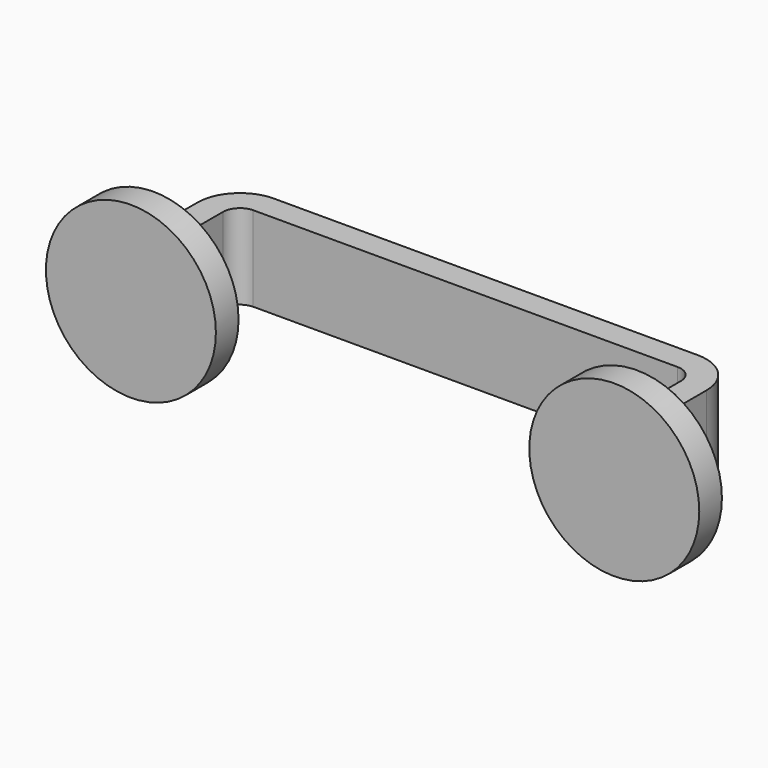
from build123d import *

# Parameters (mm, degrees)
F1_DEPTH = 30
F2_R     = 30
F3_DEPTH = 10
F4_R     = 30
F5_DEPTH = 10


# Not quite as in the source:
# - ends of sketch curves that miss each other by under 0.0002 mm in the source are joined


with BuildPart() as f1:
    # F0 (on Top) → F1 (new body)
    with BuildSketch(Plane.XY):
        with BuildLine():
            Line((-83.6328645892, 0), (-83.6328645892, -25))
            Line((-83.6328645892, -25), (-74.6328645685, -25))
            Line((-74.6328645685, -25), (-74.6328645685, 0))
            ThreePointArc((-74.6328645685, 0), (-72.9577352395, 4.1587851122), (-68.8677000121, 5.9954025783))
            Line((-68.8677000121, 5.9954025783), (80.9957853142, 5.9954025783))
            ThreePointArc((80.9957853142, 5.9954025783), (85.2384259867, 4.2380432715), (86.9957852935, -0.004597401))
            Line((86.9957852935, -0.004597401), (86.9957845889, -25))
            Line((86.9957845889, -25), (95.9957846097, -25))
            Line((95.9957846097, -25), (95.9957846097, 0))
            ThreePointArc((95.9957846097, 0), (91.6007614807, 10.603629619), (80.9957853142, 14.995402599))
            Line((80.9957853142, 14.995402599), (-69.0042146858, 14.995402599))
            ThreePointArc((-69.0042146858, 14.995402599), (-79.3699557095, 10.4744868264), (-83.6328645892, 0))
        make_face()
    extrude(amount=F1_DEPTH)

    # F2 (on face) → F3 (join)
    with BuildSketch(Plane.XZ.offset(25)):
        with Locations((-79.1328645789, 15)):
            Circle(F2_R)
    extrude(amount=F3_DEPTH)

    # F4 (on face) → F5 (join)
    with BuildSketch(Plane.XZ.offset(25)):
        with Locations((91.4957845993, 15)):
            Circle(F4_R)
    extrude(amount=F5_DEPTH)


solid = f1.part
